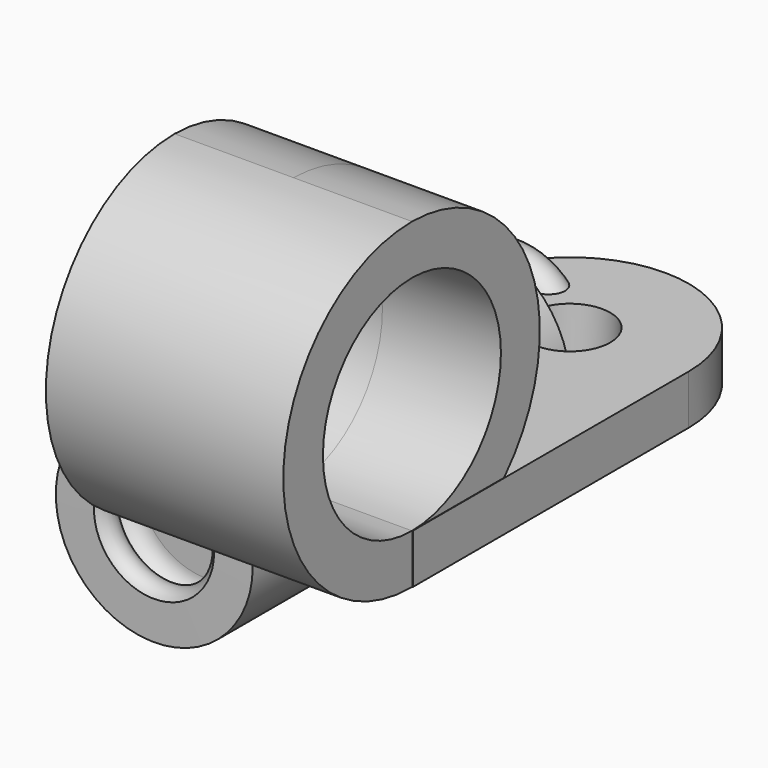
from build123d import *

# Parameters (mm, degrees)
F2_R     = 2.5908
F4_DEPTH = 3.175
F5_DEPTH = 7.5946
F6_DEPTH = 7.62


with BuildPart() as f1:
    # F0 (on Top) → F1 (revolve)
    with BuildSketch(Plane.XY):
        with BuildLine():
            Line((0, -25.4), (0, 0))
            Line((0, 0), (-3.5482933745, 0))
            ThreePointArc((-3.5482933745, 0), (-4.0205825687, 0.8574930835), (-3.5482933745, 1.7149861669))
            Line((-3.5482933745, 1.7149861669), (-2.7070879005, 1.7149861669))
            ThreePointArc((-2.7070879005, 1.7149861669), (-1.4733193675, 2.9487546999), (-2.7070879005, 4.1825232329))
            Line((-2.7070879005, 4.1825232329), (-6.309567485, 4.1623529978))
            Line((-6.309567485, 4.1623529978), (-6.309567485, -21.2779641151))
            Line((-6.309567485, -21.2779641151), (-1.9219625974, -21.2479249458))
            ThreePointArc((-1.9219625974, -21.2479249458), (-0.7142343675, -22.4556531757), (-1.9219625974, -23.6633814056))
            Line((-1.9219625974, -23.6633814056), (-2.4595375075, -23.6633814056))
            ThreePointArc((-2.4595375075, -23.6633814056), (-2.9687250789, -24.5431269868), (-2.4595375075, -25.422872568))
            Line((-2.4595375075, -25.422872568), (0, -25.4))
        make_face()
    revolve(axis=Axis((-6.309567485, -8.5578055587, 0), (0, -1, 0)))


with BuildPart() as f4:
    # F2 (on Top) → F4 (new body)
    with BuildSketch(Plane.XY):
        with BuildLine():
            Line((7.62, -22.098), (7.62, 0))
            ThreePointArc((7.62, 0), (0, 7.62), (-7.62, 0))
            Line((-7.62, 0), (-7.62, -22.098))
            Line((-7.62, -22.098), (7.62, -22.098))
        make_face()
        Circle(F2_R, mode=Mode.SUBTRACT)
    extrude(amount=F4_DEPTH)


with BuildPart() as f5:
    # F3 (on Right) → F5 (new body)
    with BuildSketch(Plane.YZ):
        with BuildLine():
            Line((-22.1333019435, 17.4498), (-22.1333019435, 20.6248))
            ThreePointArc((-22.1333019435, 20.6248), (-32.4457019435, 10.3124), (-22.1333019435, 0))
            Line((-22.1333019435, 0), (-22.1333019435, 3.175))
            ThreePointArc((-22.1333019435, 3.175), (-29.2707019435, 10.3124), (-22.1333019435, 17.4498))
        make_face()
        with BuildLine():
            ThreePointArc((-22.1333019435, 0), (-11.8989743379, 10.3124), (-22.1333019435, 20.6248))
            Line((-22.1333019435, 20.6248), (-22.1333019435, 17.4498))
            ThreePointArc((-22.1333019435, 17.4498), (-15.0133552942, 10.3124), (-22.1333019435, 3.175))
            Line((-22.1333019435, 3.175), (-22.1333019435, 0))
        make_face()
    extrude(amount=F5_DEPTH)

    # F5_face (on face) + F3 (on Right) → F6 (join)
    with BuildSketch(Plane(origin=(0, -22.2003075757, 10.3124), x_dir=(0, 1, 0), z_dir=(-1, 0, 0))):
        with BuildLine():
            ThreePointArc((0.0670056321, 10.3124), (-10.2453943679, 0), (0.0670056321, -10.3124))
            ThreePointArc((0.0670056321, -10.3124), (10.3013332378, 0), (0.0670056321, 10.3124))
        make_face()
        with BuildLine():
            ThreePointArc((0.0670056321, -7.1374), (-7.0703943679, 0), (0.0670056321, 7.1374))
            ThreePointArc((0.0670056321, 7.1374), (7.1869522815, 0), (0.0670056321, -7.1374))
        make_face(mode=Mode.SUBTRACT)
    with BuildSketch(Plane.YZ):
        with BuildLine():
            Line((-22.1333019435, 17.4498), (-22.1333019435, 20.6248))
            ThreePointArc((-22.1333019435, 20.6248), (-32.4457019435, 10.3124), (-22.1333019435, 0))
            Line((-22.1333019435, 0), (-22.1333019435, 3.175))
            ThreePointArc((-22.1333019435, 3.175), (-29.2707019435, 10.3124), (-22.1333019435, 17.4498))
        make_face()
        with BuildLine():
            ThreePointArc((-22.1333019435, 0), (-11.8989743379, 10.3124), (-22.1333019435, 20.6248))
            Line((-22.1333019435, 20.6248), (-22.1333019435, 17.4498))
            ThreePointArc((-22.1333019435, 17.4498), (-15.0133552942, 10.3124), (-22.1333019435, 3.175))
            Line((-22.1333019435, 3.175), (-22.1333019435, 0))
        make_face()
    extrude(amount=F6_DEPTH, dir=(-1, 0, 0))


solid = Compound([f1.part, f4.part, f5.part])
